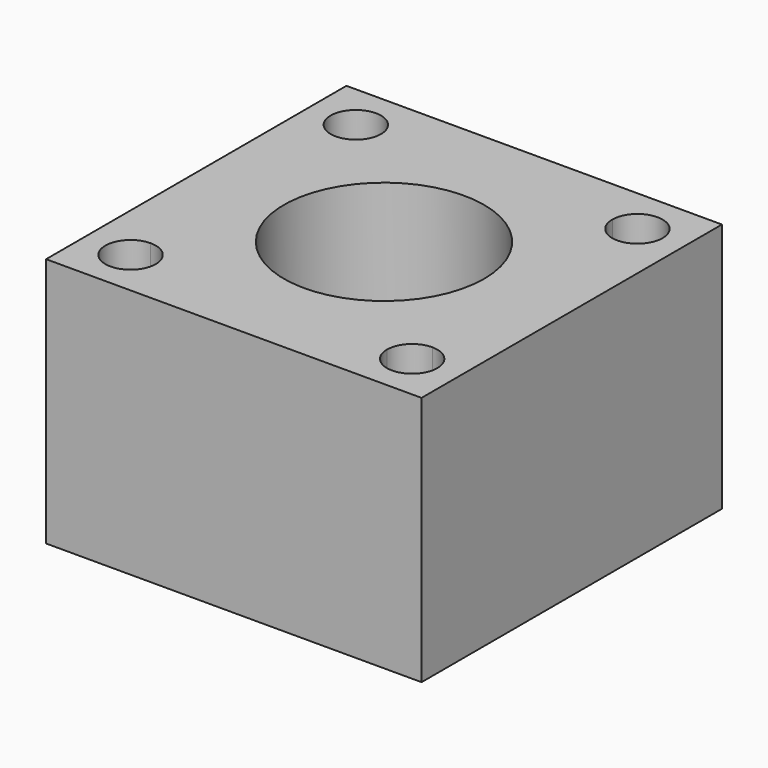
from build123d import *

# Parameters (mm, degrees)
F0_W     = 25.4
F0_H     = 14.2875
F1_DEPTH = 25.4
F2_R     = 10.16
F3_DEPTH = 25.401
F5_DEPTH = 25.401


# Not quite as in the source:
# - a feature names something its author has since deleted; it is built from what else it names


with BuildPart() as f1:
    # F0 (on Top) → F1 (new body)
    with BuildSketch(Plane.XY):
        with Locations((-34.7179355979, 53.2439169049)):
            Rectangle(F0_W, F0_H)
        Polygon((-22.0179355979, 46.1001669049), (-47.4179355979, 46.1001669049), (-47.4179355979, -30.0998330951), (-22.0179355979, -30.0998330951), (54.1820644021, -30.0998330951), (54.1820644021, 46.1001669049), align=None)
        with Locations((-34.7179355979, -37.2435830951)):
            Rectangle(F0_W, F0_H)
    extrude(amount=F1_DEPTH)

    # F2 (on face) → F3 (cut, through all)
    with BuildSketch(Plane.XY.offset(25.4)):
        with Locations((35.1320644021, 8.0001669049)):
            Circle(F2_R)
        with BuildLine():
            Line((23.3972644021, 22.2876669049), (20.8445644021, 22.2876669049))
            Line((20.8445644021, 22.2876669049), (20.8445644021, 19.7349669049))
            ThreePointArc((20.8445644021, 19.7349669049), (22.6495958824, 20.4826354246), (23.3972644021, 22.2876669049))
        make_face()
        with BuildLine():
            Line((20.8445644021, 19.7349669049), (20.8445644021, 22.2876669049))
            Line((20.8445644021, 22.2876669049), (23.3972644021, 22.2876669049))
            ThreePointArc((23.3972644021, 22.2876669049), (19.0395329218, 24.0926983853), (20.8445644021, 19.7349669049))
        make_face()
        with BuildLine():
            ThreePointArc((51.9722644021, 22.2876669049), (49.4195644021, 24.8403669049), (46.8668644021, 22.2876669049))
            Line((46.8668644021, 22.2876669049), (49.4195644021, 22.2876669049))
            Line((49.4195644021, 22.2876669049), (49.4195644021, 19.7349669049))
            ThreePointArc((49.4195644021, 19.7349669049), (51.2245958824, 20.4826354246), (51.9722644021, 22.2876669049))
        make_face()
        with BuildLine():
            Line((49.4195644021, 22.2876669049), (46.8668644021, 22.2876669049))
            ThreePointArc((46.8668644021, 22.2876669049), (47.6145329218, 20.4826354246), (49.4195644021, 19.7349669049))
            Line((49.4195644021, 19.7349669049), (49.4195644021, 22.2876669049))
        make_face()
        with BuildLine():
            Line((49.4195644021, -6.2873330951), (49.4195644021, -3.7346330951))
            ThreePointArc((49.4195644021, -3.7346330951), (47.6145329218, -4.4823016147), (46.8668644021, -6.2873330951))
            Line((46.8668644021, -6.2873330951), (49.4195644021, -6.2873330951))
        make_face()
        with BuildLine():
            ThreePointArc((51.9722644021, -6.2873330951), (51.2245958824, -4.4823016147), (49.4195644021, -3.7346330951))
            Line((49.4195644021, -3.7346330951), (49.4195644021, -6.2873330951))
            Line((49.4195644021, -6.2873330951), (46.8668644021, -6.2873330951))
            ThreePointArc((46.8668644021, -6.2873330951), (49.4195644021, -8.8400330951), (51.9722644021, -6.2873330951))
        make_face()
        with BuildLine():
            ThreePointArc((23.3972644021, -6.2873330951), (22.6495958824, -4.4823016147), (20.8445644021, -3.7346330951))
            Line((20.8445644021, -3.7346330951), (20.8445644021, -6.2873330951))
            Line((20.8445644021, -6.2873330951), (23.3972644021, -6.2873330951))
        make_face()
        with BuildLine():
            Line((20.8445644021, -6.2873330951), (20.8445644021, -3.7346330951))
            ThreePointArc((20.8445644021, -3.7346330951), (19.0395329218, -8.0923645754), (23.3972644021, -6.2873330951))
            Line((23.3972644021, -6.2873330951), (20.8445644021, -6.2873330951))
        make_face()
    extrude(amount=-F3_DEPTH, mode=Mode.SUBTRACT)

    # F4 (on face) → F5 (cut, through all)
    with BuildSketch(Plane.XY.offset(25.4)):
        Polygon((54.1820644021, -30.0998330951), (54.1820644021, -11.0498330951), (16.0820644021, -11.0498330951), (16.0820644021, 27.0501669049), (54.1820644021, 27.0501669049), (54.1820644021, 46.1001669049), (-22.0179355979, 46.1001669049), (-22.0179355979, 60.3876669049), (-47.4179355979, 60.3876669049), (-47.4179355979, -44.3873330951), (-22.0179355979, -44.3873330951), (-22.0179355979, -30.0998330951), align=None)
    extrude(amount=-F5_DEPTH, mode=Mode.SUBTRACT)


solid = f1.part
